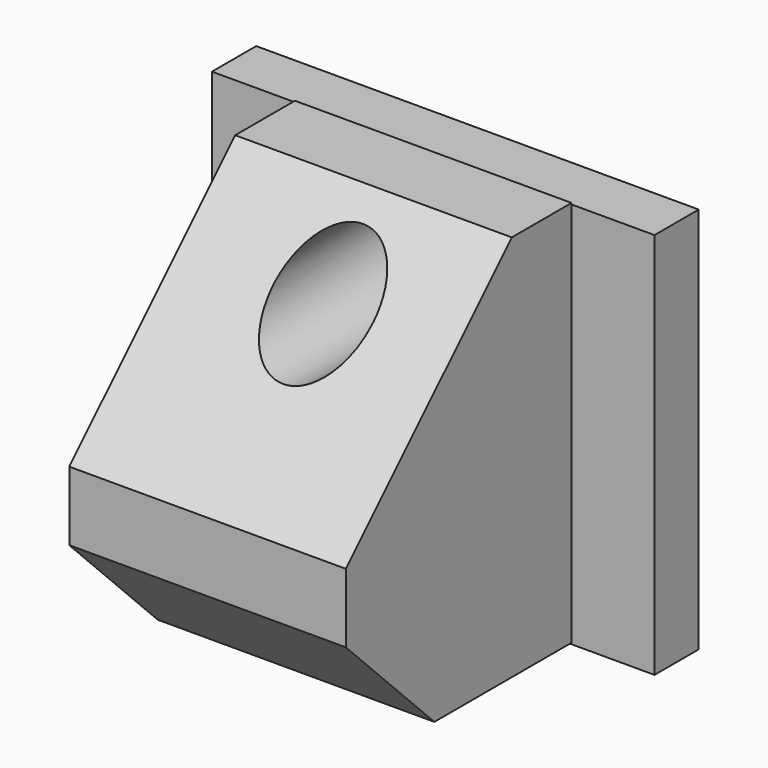
from build123d import *

# Parameters (mm, degrees)
F0_W        = 320
F0_H        = 280
F1_DEPTH    = 40
F2_W        = 200
F2_H        = 0.9724124948
F2_H_2      = 279.0275875052
F2_R        = 36.2270476268
F3_DEPTH    = 204
F4_T1_DEPTH = 971.5048963898
F5_SIZE     = 80


# Not quite as in the source:
# - a fillet or chamfer that OpenCascade refuses, or shapes differently, is made with other operations: its cross-section is extruded or revolved along the edge and cut away or added
# - a feature of the source that left no trace in its solid (it failed there, or was rolled back) is left out


with BuildPart() as f1:
    # F0 (on Front) → F1 (new body)
    with BuildSketch(Plane.XZ):
        with Locations((0.0898987055, 70.5860536863)):
            Rectangle(F0_W, F0_H)
    extrude(amount=F1_DEPTH)


with BuildPart() as f3:
    # F2 (on face) → F3 (new body)
    with BuildSketch(Plane.XZ.offset(40)):
        with Locations((0.0898987055, 211.0722599337)):
            Rectangle(F2_W, F2_H)
        with Locations((0.0898987055, 71.0722599337)):
            Rectangle(F2_W, F2_H_2)
        with Locations((5.2852756344, 159.5223546028)):
            Circle(F2_R, mode=Mode.SUBTRACT)
    extrude(amount=F3_DEPTH)

    # F4: chamfer of 150 on 1 edges, made by hand

    # F4_s2 → F4_t1 (cut)
    with BuildSketch(Plane.YZ.offset(-485.6625494894)):
        Polygon((-94, 211.5584661812), (-244, 61.5584661812), (-244, 211.5584661812), align=None)
    extrude(amount=F4_T1_DEPTH, mode=Mode.SUBTRACT)

    # F5
    f5_edges = [f3.edges().sort_by_distance(p)[0] for p in [
        (0.089899, -244, -68.441534),
    ]]
    chamfer(f5_edges, length=F5_SIZE)


solid = Compound([f1.part, f3.part])
